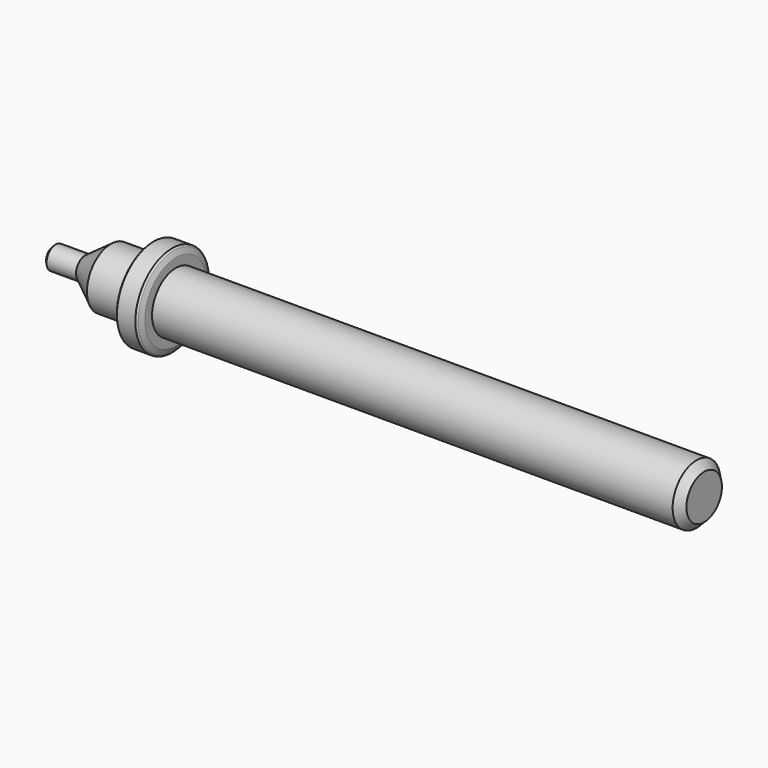
from build123d import *

# Parameters (mm, degrees)
F0_W    = 14
F0_H    = 3.9
F2_SIZE = 0.5
F3_SIZE = 0.1
F4_SIZE = 0.3


# Not quite as in the source:
# - a fillet or chamfer that OpenCascade refuses, or shapes differently, is made with other operations: its cross-section is extruded or revolved along the edge and cut away or added


with BuildPart() as f1:
    # F0 (on Front) → F1 (revolve)
    with BuildSketch(Plane.XZ):
        Polygon((0, 1.5), (0, 0), (71, 0), (71, 3.9), (16, 3.9), (16, 6), (13, 6), (13, 3.9), (7.5, 3.9), (4.1531170718, 1.5), align=None)
        with Locations((78, 1.95)):
            Rectangle(F0_W, F0_H)
    revolve(axis=Axis((35.5, 0, 0), (1, 0, 0)))

    # F2
    f2_edges = [f1.edges().sort_by_distance(p)[0] for p in [
        (16, 0, -6),
    ]]
    chamfer(f2_edges, length=F2_SIZE)

    # F3
    f3_edges = [f1.edges().sort_by_distance(p)[0] for p in [
        (13, 0, -6),
    ]]
    chamfer(f3_edges, length=F3_SIZE)

    # F4
    f4_edges = [f1.edges().sort_by_distance(p)[0] for p in [
        (0, 0, -1.5),
    ]]
    chamfer(f4_edges, length=F4_SIZE)

    # F5: chamfer of 1 on 2 edges, made by hand

    # F5_s1 → F5_t2 (revolve, cut)
    with BuildSketch(Plane.XZ):
        Polygon((15.7071067812, 5.7928932188), (16, 5.0857864376), (16, 5.5), align=None)
    revolve(axis=Axis((16, 0, 0), (1, 0, 0)), mode=Mode.SUBTRACT)

    # F5_s3 → F5_t4 (revolve, cut)
    with BuildSketch(Plane.XZ):
        Polygon((84, 3.9), (85, 2.9), (85, 3.9), align=None)
    revolve(axis=Axis((85, 0, 0), (1, 0, 0)), mode=Mode.SUBTRACT)


solid = f1.part
